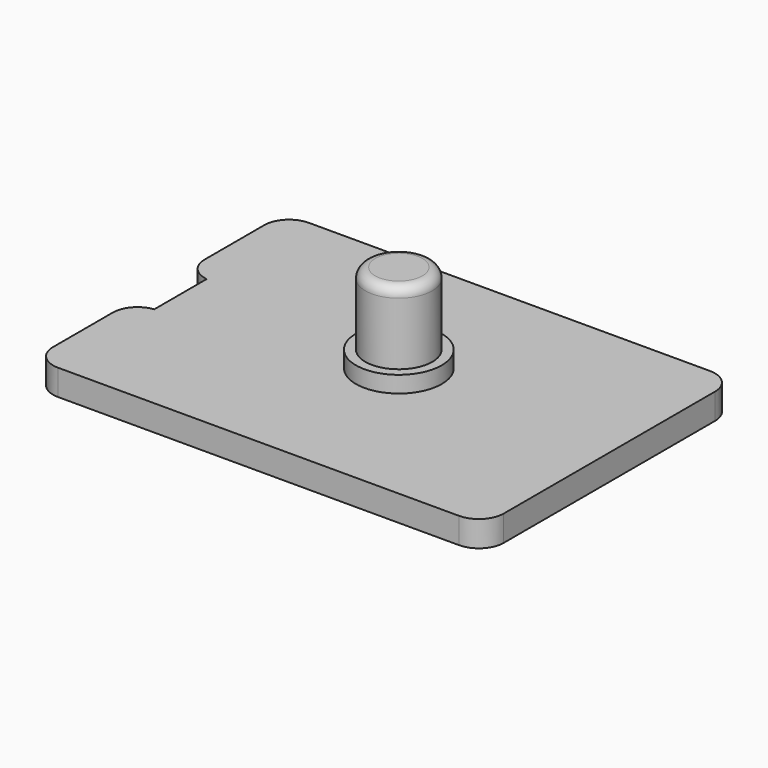
from build123d import *

# Parameters (mm, degrees)
F1_DEPTH    = 2.6
F2_T1_DEPTH = 15.1
F2_T3_DEPTH = 15.009673646
F3_R        = 4.32
F4_DEPTH    = 1.66
F5_R        = 3.375
F6_DEPTH    = 7.3
F7_R        = 1


# Not quite as in the source:
# - a fillet or chamfer that OpenCascade refuses, or shapes differently, is made with other operations: its cross-section is extruded or revolved along the edge and cut away or added


with BuildPart() as f1:
    # F0 (on Top) → F1 (new body)
    with BuildSketch(Plane.XY):
        Polygon((0, 12.5), (0, 0), (45.4, 0), (45.4, 31.6), (0, 31.6), (0, 19.1), (2.2, 19.1), (2.2, 12.5), align=None)
    extrude(amount=F1_DEPTH)

    # F2: fillet of radius 2.5 on 6 edges, made by hand

    # F2_s2 → F2_t1 (cut)
    with BuildSketch(Plane.XY.offset(-6.25)):
        with BuildLine():
            ThreePointArc((45.4, 29.1), (44.667766953, 30.867766953), (42.9, 31.6))
            Line((42.9, 31.6), (45.4, 31.6))
            Line((45.4, 31.6), (45.4, 29.1))
        make_face()
        with BuildLine():
            ThreePointArc((2.5, 31.6), (0.732233047, 30.867766953), (0, 29.1))
            Line((0, 29.1), (0, 31.6))
            Line((0, 31.6), (2.5, 31.6))
        make_face()
        with BuildLine():
            ThreePointArc((42.9, 0), (44.667766953, 0.732233047), (45.4, 2.5))
            Line((45.4, 2.5), (45.4, 0))
            Line((45.4, 0), (42.9, 0))
        make_face()
        with BuildLine():
            ThreePointArc((0, 2.5), (0.732233047, 0.732233047), (2.5, 0))
            Line((2.5, 0), (0, 0))
            Line((0, 0), (0, 2.5))
        make_face()
    extrude(amount=F2_T1_DEPTH, mode=Mode.SUBTRACT)

    # F2_s4 → F2_t3 (cut)
    with BuildSketch(Plane.XY.offset(-6.204836823)):
        with BuildLine():
            ThreePointArc((0, 21.5819347292), (0.6291713066, 19.923622334), (2.2, 19.1))
            Line((2.2, 19.1), (0, 19.1))
            Line((0, 19.1), (0, 21.5819347292))
        make_face()
        with BuildLine():
            ThreePointArc((0, 10.0180652708), (0.6291713066, 11.676377666), (2.2, 12.5))
            Line((2.2, 12.5), (0, 12.5))
            Line((0, 12.5), (0, 10.0180652708))
        make_face()
    extrude(amount=F2_T3_DEPTH, mode=Mode.SUBTRACT)

    # F3 (on face) → F4 (join)
    with BuildSketch(Plane.XY.offset(2.6)):
        with Locations((23.49, 16.68)):
            Circle(F3_R)
    extrude(amount=F4_DEPTH)

    # F5 (on face) → F6 (join)
    with BuildSketch(Plane.XY.offset(4.26)):
        with Locations((23.49, 16.68)):
            Circle(F5_R)
    extrude(amount=F6_DEPTH)

    # F7
    f7_edges = [f1.edges().sort_by_distance(p)[0] for p in [
        (20.115, 16.68, 11.56),
    ]]
    fillet(f7_edges, radius=F7_R)


solid = f1.part
